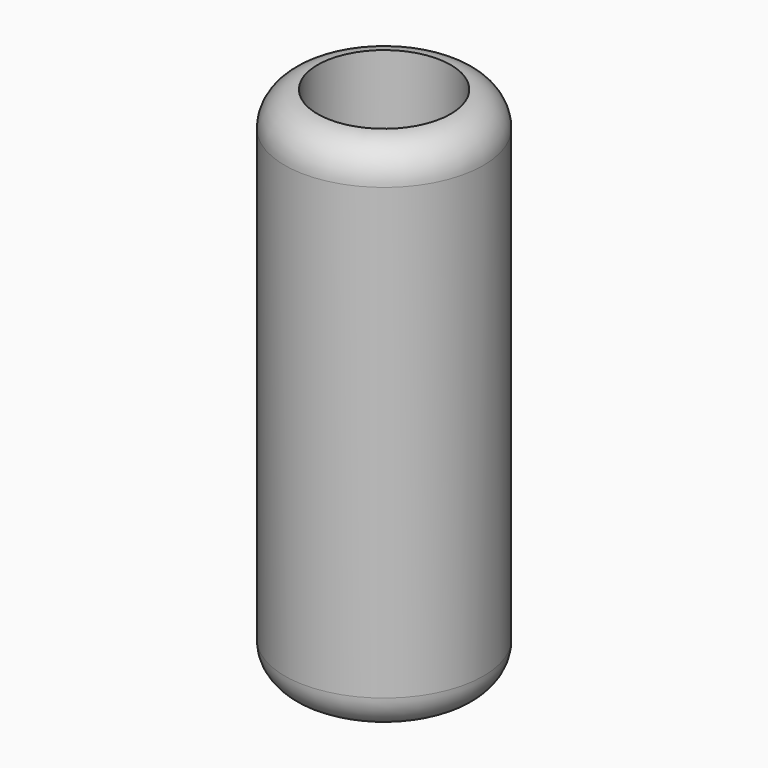
from build123d import *

# Parameters (mm, degrees)
F0_R     = 5.75
F0_R_2   = 3.85
F0_R_3   = 3.6
F1_DEPTH = 30
F2_DEPTH = 15
F3_START = 15
F3_DEPTH = 15


# Not quite as in the source:
# - a fillet or chamfer that OpenCascade refuses, or shapes differently, is made with other operations: its cross-section is extruded or revolved along the edge and cut away or added
# - a feature names something its author has since deleted; it is built from what else it names


with BuildPart() as f1:
    # F0 (on Top) → F1 (new body)
    with BuildSketch(Plane.XY):
        Circle(F0_R)
        Circle(F0_R_2, mode=Mode.SUBTRACT)
        Circle(F0_R_2)
        Circle(F0_R_3, mode=Mode.SUBTRACT)
        Circle(F0_R_3)
    extrude(amount=F1_DEPTH)

    # F0 (on Top) → F2 (cut)
    with BuildSketch(Plane.XY):
        Circle(F0_R_3)
    extrude(amount=F2_DEPTH, mode=Mode.SUBTRACT)

    # F0 (on Top) → F3 (cut)
    with BuildSketch(Plane.XY.offset(F3_START)):
        Circle(F0_R_2)
        Circle(F0_R_3, mode=Mode.SUBTRACT)
        Circle(F0_R_3)
    extrude(amount=F3_DEPTH, mode=Mode.SUBTRACT)

    # F4: fillet of radius 2 on 2 edges, made by hand

    # F4_s1 → F4_t2 (revolve, cut)
    with BuildSketch(Plane.XZ):
        with BuildLine():
            ThreePointArc((5.75, 28.0025015645), (5.1991376746, 29.3809064397), (3.85, 30))
            Line((3.85, 30), (5.75, 30))
            Line((5.75, 30), (5.75, 28.0025015645))
        make_face()
    revolve(axis=Axis((0, 0, 30), (0, 0, 1)), mode=Mode.SUBTRACT)

    # F4_s3 → F4_t4 (revolve, cut)
    with BuildSketch(Plane.XZ):
        with BuildLine():
            ThreePointArc((5.75, 2), (5.1642135624, 0.5857864376), (3.75, 0))
            Line((3.75, 0), (5.75, 0))
            Line((5.75, 0), (5.75, 2))
        make_face()
    revolve(axis=Axis((0, 0, 0), (0, 0, 1)), mode=Mode.SUBTRACT)


solid = f1.part
